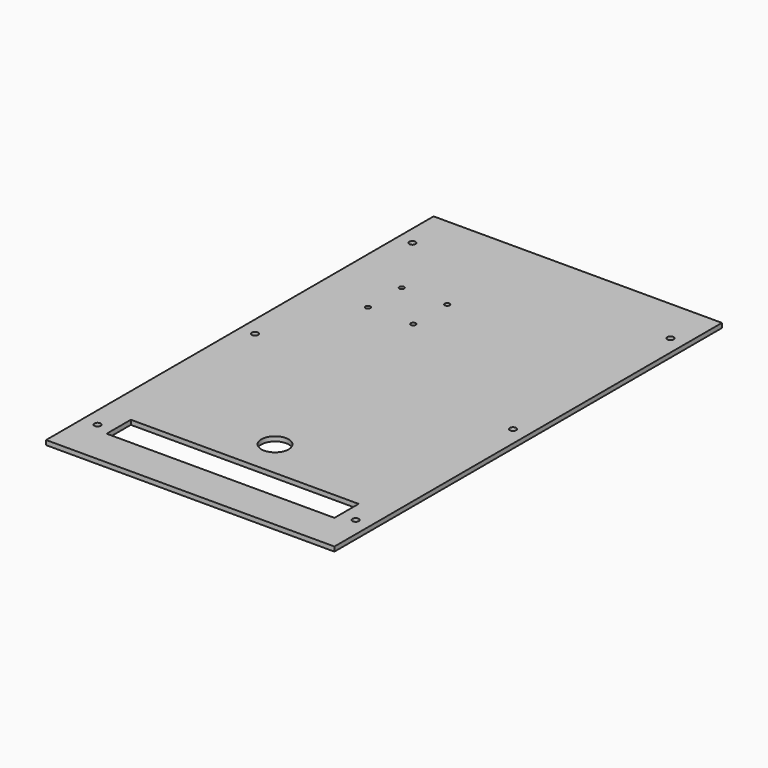
from build123d import *

# Parameters (mm, degrees)
F1_W      = 190.5
F1_H      = 320
F2_DEPTH  = 3
F4_D      = 4.2
F4_DEPTH  = 4
F4_TIP    = 1.2618073
F6_D      = 3.2
F6_DEPTH  = 4
F6_TIP    = 0.9613769904
F7_W      = 150.5
F7_H      = 20
F8_DEPTH  = 25
F9_R      = 9
F10_DEPTH = 3


# Not quite as in the source:
# - a pattern or mirror of a feature is missing from the dataset's text; its kind, count and spacing are read off the source's solid


with BuildPart() as f2:
    # F1 (on Top) → F2 (new body)
    with BuildSketch(Plane.XY):
        Rectangle(F1_W, F1_H)
    extrude(amount=F2_DEPTH)

    # F4
    with Locations(Plane.XY.offset(3)):
        with Locations((-85.25, 130), (-85.25, 0), (-85.25, -130)):
            f4 = Hole(F4_D / 2, depth=F4_DEPTH)
            with Locations((0, 0, -(F4_DEPTH + F4_TIP / 2))):  # 118° drill point
                Cone(0, F4_D / 2, F4_TIP, mode=Mode.SUBTRACT)

    # F4_copies: F4 across plane
    add(f4.mirror(Plane(origin=(0, 0, 0), x_dir=(0, 0, 1), z_dir=(1, 0, 0))), mode=Mode.SUBTRACT)

    # F6
    with Locations(Plane.XY.offset(3)):
        with Locations((-58.25, 87.5), (-58.25, 59.5), (-28.25, 59.5), (-28.25, 87.5)):
            Hole(F6_D / 2, depth=F6_DEPTH)
            with Locations((0, 0, -(F6_DEPTH + F6_TIP / 2))):  # 118° drill point
                Cone(0, F6_D / 2, F6_TIP, mode=Mode.SUBTRACT)

    # F7 (on face) → F8 (cut)
    with BuildSketch(Plane.XY.offset(3)):
        with Locations((0, -125)):
            Rectangle(F7_W, F7_H)
    extrude(amount=-F8_DEPTH, mode=Mode.SUBTRACT)

    # F9 (on face) → F10 (cut, through all)
    with BuildSketch(Plane(origin=(0, 0, 0), x_dir=(1, 0, 0), z_dir=(0, 0, -1))):
        with Locations((0, 90)):
            Circle(F9_R)
    extrude(amount=-F10_DEPTH, mode=Mode.SUBTRACT)


solid = f2.part
